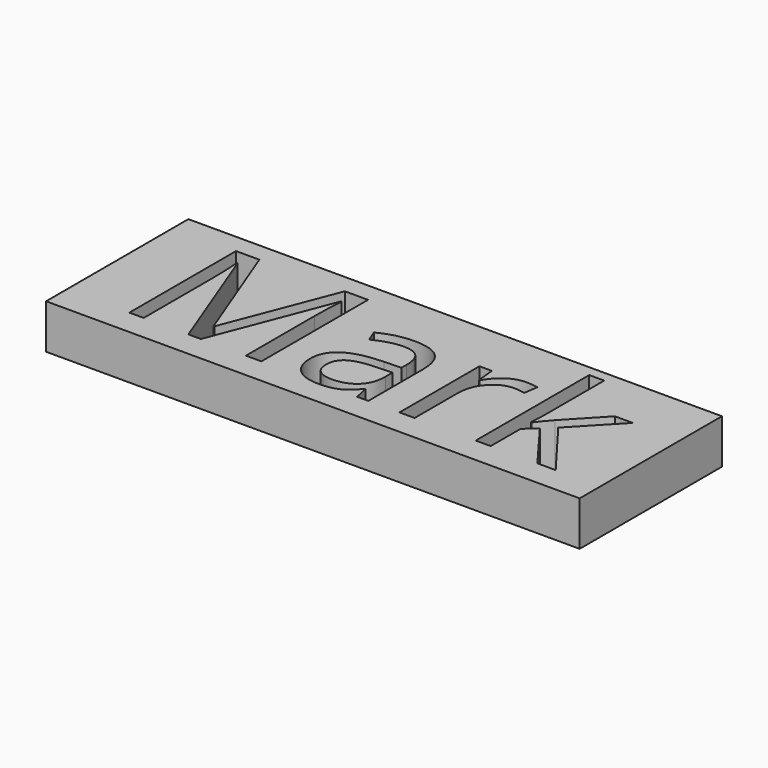
from build123d import *

# Parameters (mm, degrees)
F0_W         = 60
F0_H         = 20
F1_DEPTH     = 5
F2_TEXT_SIZE = 20.995997638
F3_DEPTH     = 5.001


# Not quite as in the source:
# - Text() gives the source's letters only with a copy of the font that has no kerning and outlines rounded to 1/6400 em; it was checked with that copy


with BuildPart() as f1:
    # F0 (on Top) → F1 (new body)
    with BuildSketch(Plane.XY):
        Rectangle(F0_W, F0_H)
    extrude(amount=F1_DEPTH)

    # F2 (on face) → F3 (cut, through all)
    with BuildSketch(Plane.XY.offset(5)):
        with Locations((-25, -7.1171182993)):
            Text('Mark', F2_TEXT_SIZE, font='Open Sans', text_align=(TextAlign.LEFT, TextAlign.BOTTOM))
    extrude(amount=-F3_DEPTH, mode=Mode.SUBTRACT)


solid = f1.part
